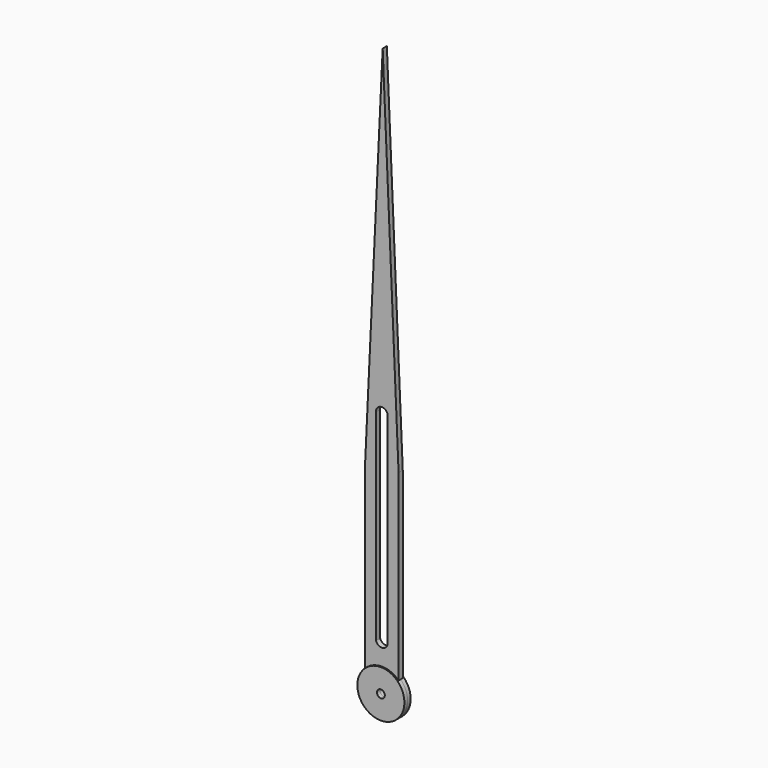
from build123d import *

# Parameters (mm, degrees)
F0_R     = 1.5
F1_DEPTH = 1.5
F2_DEPTH = 1


# Not quite as in the source:
# - a feature names something its author has since deleted; it is built from what else it names


with BuildPart() as f1:
    # F0 (on Front) → F1 (new body, symmetric)
    with BuildSketch(Plane.XZ):
        with BuildLine():
            ThreePointArc((-26.4131706208, -37.9566435516), (-23.481364387, -52.6302208163), (-11.041955635, -44.3133423492))
            ThreePointArc((-11.041955635, -44.3133423492), (-11.7250771679, -40.8739335972), (-13.6707406491, -37.9566435516))
            ThreePointArc((-13.6707406491, -37.9566435516), (-20.041955635, -35.3133423492), (-26.4131706208, -37.9566435516))
        make_face()
        with Locations((-20.041955635, -44.3133423492)):
            Circle(F0_R, mode=Mode.SUBTRACT)
    extrude(amount=F1_DEPTH, both=True)

    # F0 (on Front) → F2 (join, symmetric)
    with BuildSketch(Plane.XZ):
        with BuildLine():
            ThreePointArc((-26.4131706208, -37.9566435516), (-20.041955635, -35.3133423492), (-13.6707406491, -37.9566435516))
            Line((-13.6707406491, -37.9566435516), (-13.6707406491, 32.0433564484))
            Line((-13.6707406491, 32.0433564484), (-19.7518970817, 172.8046387434))
            Line((-19.7518970817, 172.8046387434), (-26.4131706208, 32.0433564484))
            Line((-26.4131706208, 32.0433564484), (-26.4131706208, -37.9566435516))
        make_face()
        with BuildLine():
            ThreePointArc((-17.8331751789, -27.2142183483), (-20.0164253794, -28.9654707243), (-22.2972274289, -27.3433091007))
            Line((-22.2972274289, -27.3433091007), (-22.2972274289, 49.6566908993))
            ThreePointArc((-22.2972274289, 49.6566908993), (-20.1316401752, 52.0187408382), (-17.8331751789, 49.7857816517))
            Line((-17.8331751789, 49.7857816517), (-17.8331751789, -27.2142183483))
        make_face(mode=Mode.SUBTRACT)
    extrude(amount=F2_DEPTH, both=True)


solid = f1.part
